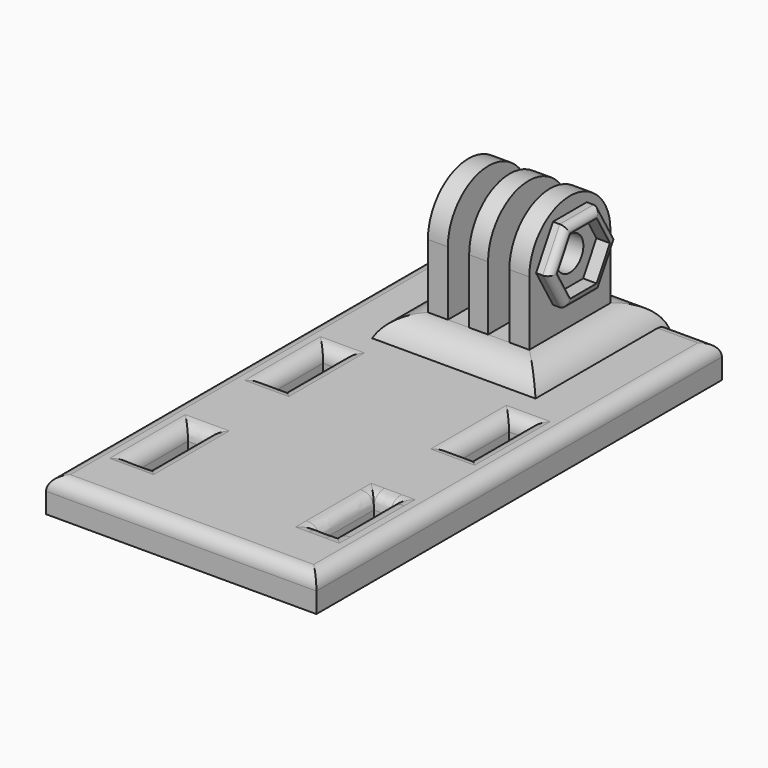
from build123d import *

# Parameters (mm, degrees)
F0_W           = 15
F0_H           = 3
F1_DEPTH       = 15
F2_DEPTH       = 3
F3_DEPTH       = 3
F4_DEPTH       = 2
F5_DEPTH       = 3
F6_DEPTH       = 12
F7_D           = 5
F7_DEPTH       = 15
F7_TIP         = 1.5021515476
F9_W           = 3.15
F9_H           = 15
F10_DEPTH      = 17
F11_R          = 1
F12_W          = 12.5
F12_H          = 12.5
F13_DEPTH      = 5
F14_T1_DEPTH   = 2.5
F14_T3_DEPTH   = 10
F14_T9_DEPTH   = 15
F14_T13_DEPTH  = 7.5
F14_T20_DEPTH  = 7.5
F14_T24_DEPTH  = 15
F14_T31_DEPTH  = 15
F14_T35_DEPTH  = 7.5
F14_T42_DEPTH  = 15
F14_T46_DEPTH  = 7.5
F15_R          = 2
F17_W          = 20
F17_H          = 12.5
F17_W_2        = 5
F18_DEPTH      = 3
F18_DEPTH_BACK = 2
F19_R          = 4.99999


# Not quite as in the source:
# - a fillet or chamfer that OpenCascade refuses, or shapes differently, is made with other operations: its cross-section is extruded or revolved along the edge and cut away or added
# - a fillet or chamfer is up to 0.001 mm smaller than in the source, because OpenCascade refuses the exact size


with BuildPart() as f1:
    # F0 (on Right) → F1 (new body)
    with BuildSketch(Plane.YZ):
        with Locations((0, 1.5)):
            Rectangle(F0_W, F0_H)
    extrude(amount=-F1_DEPTH)

    # F0 (on Right) → F2 (join)
    with BuildSketch(Plane.YZ):
        with BuildLine():
            Line((-7.5, 12.5), (-7.5, 3))
            Line((-7.5, 3), (7.5, 3))
            Line((7.5, 3), (7.5, 12.5))
            ThreePointArc((7.5, 12.5), (0, 20), (-7.5, 12.5))
        make_face()
        Polygon((-6.25, 12.5), (-3.125, 17.9126587737), (3.125, 17.9126587737), (6.25, 12.5), (3.125, 7.0873412263), (-3.125, 7.0873412263), align=None, mode=Mode.SUBTRACT)
    extrude(amount=-F2_DEPTH)

    # F0 (on Right) → F3 (join)
    with BuildSketch(Plane.YZ):
        Polygon((3.125, 17.9126587737), (-3.125, 17.9126587737), (-6.25, 12.5), (-3.125, 7.0873412263), (3.125, 7.0873412263), (6.25, 12.5), align=None)
        Polygon((-4.9074772881, 12.5), (-2.4537386441, 16.75), (2.4537386441, 16.75), (4.9074772881, 12.5), (2.4537386441, 8.25), (-2.4537386441, 8.25), align=None, mode=Mode.SUBTRACT)
    extrude(amount=-F3_DEPTH)

    # F0 (on Right) → F4 (join)
    with BuildSketch(Plane.YZ):
        Polygon((3.125, 17.9126587737), (-3.125, 17.9126587737), (-6.25, 12.5), (-3.125, 7.0873412263), (3.125, 7.0873412263), (6.25, 12.5), align=None)
        Polygon((-4.9074772881, 12.5), (-2.4537386441, 16.75), (2.4537386441, 16.75), (4.9074772881, 12.5), (2.4537386441, 8.25), (-2.4537386441, 8.25), align=None, mode=Mode.SUBTRACT)
    extrude(amount=F4_DEPTH)

    # F0 (on Right) → F5 (join)
    with BuildSketch(Plane.YZ):
        Polygon((2.4537386441, 16.75), (-2.4537386441, 16.75), (-4.9074772881, 12.5), (-2.4537386441, 8.25), (2.4537386441, 8.25), (4.9074772881, 12.5), align=None)
    extrude(amount=-F5_DEPTH)

    # F6 (add): a face of the model
    f6_faces = [f1.faces().sort_by_distance(p)[0] for p in [
        (-3, 0, 10.7862789639),
    ]]
    extrude(f6_faces, amount=F6_DEPTH)

    # F7
    with Locations(Plane.YZ):
        with Locations((0, 12.5)):
            Hole(F7_D / 2, depth=F7_DEPTH)
            with Locations((0, 0, -(F7_DEPTH + F7_TIP / 2))):  # 118° drill point
                Cone(0, F7_D / 2, F7_TIP, mode=Mode.SUBTRACT)

    # F9 (on offset) → F10 (cut)
    with BuildSketch(Plane.XY.offset(20)):
        with Locations((-10.475, 0)):
            Rectangle(F9_W, F9_H)
        with Locations((-4.525, 0)):
            Rectangle(F9_W, F9_H)
    extrude(amount=-F10_DEPTH, mode=Mode.SUBTRACT)

    # F11
    f11_edges = [f1.edges().sort_by_distance(p)[0] for p in [
        (2, -4.6875, 9.793671),
        (2, 0, 7.087341),
        (2, -4.6875, 15.206329),
        (2, 0, 17.912659),
        (2, 4.6875, 15.206329),
        (2, 4.6875, 9.793671),
    ]]
    fillet(f11_edges, radius=F11_R)


with BuildPart() as f13:
    # F12 (on face) → F13 (new body)
    with BuildSketch(Plane(origin=(0, 0, 0), x_dir=(1, 0, 0), z_dir=(0, 0, -1))):
        Polygon((-27.5, -12.5), (0, -12.5), (0, 0), (0, 62.5), (-20, 62.5), (-20, 52.5), (-20, 42.5), (-20, 27.5), (-20, 17.5), (-22.5, 17.5), (-27.5, 17.5), (-27.5, 0), align=None)
        with Locations((6.25, -6.25)):
            Rectangle(F12_W, F12_H)
        Polygon((0, 62.5), (0, 0), (12.5, 0), (12.5, 17.5), (7.5, 17.5), (5, 17.5), (5, 27.5), (5, 42.5), (5, 52.5), (5, 62.5), align=None)
        Polygon((-27.5, 42.5), (-27.5, 17.5), (-22.5, 17.5), (-22.5, 27.5), (-20, 27.5), (-20, 42.5), (-22.5, 42.5), align=None)
        Polygon((-20, 52.5), (-20, 62.5), (-27.5, 62.5), (-27.5, 42.5), (-22.5, 42.5), (-22.5, 52.5), align=None)
        Polygon((12.5, 62.5), (5, 62.5), (5, 52.5), (7.5, 52.5), (12.5, 52.5), align=None)
        Polygon((7.5, 17.5), (12.5, 17.5), (12.5, 52.5), (7.5, 52.5), (7.5, 42.5), (5, 42.5), (5, 27.5), (7.5, 27.5), align=None)
    extrude(amount=F13_DEPTH)

    # F14: fillet of radius 2 on 4 edges, made by hand

    # F14_s2 → F14_t1 (cut)
    with BuildSketch(Plane.YZ.offset(5)):
        with BuildLine():
            add(Edge.make_bspline(
                [(-52.5, -2), (-52.5, 0), (-54.5, 0)],
                knots=[0, 0, 0, 1, 1, 1], degree=2, weights=[1, 1, 1]))
            Line((-54.5, 0), (-52.5, 0))
            Line((-52.5, 0), (-52.5, -2))
        make_face()
        with BuildLine():
            add(Edge.make_bspline(
                [(-42.5, -2), (-42.5, 0), (-40.5, 0)],
                knots=[0, 0, 0, 1, 1, 1], degree=2, weights=[1, 1, 1]))
            Line((-40.5, 0), (-42.5, 0))
            Line((-42.5, 0), (-42.5, -2))
        make_face()
    extrude(amount=F14_T1_DEPTH, mode=Mode.SUBTRACT)

    # F14_s4 → F14_t3 (cut)
    with BuildSketch(Plane.XZ.offset(42.5)):
        with BuildLine():
            add(Edge.make_bspline(
                [(7.5, -2), (7.5, 0), (9.5, 0)],
                knots=[0, 0, 0, 1, 1, 1], degree=2, weights=[1, 1, 1]))
            Line((9.5, 0), (7.5, 0))
            Line((7.5, 0), (7.5, -2))
        make_face()
        with BuildLine():
            add(Edge.make_bspline(
                [(5, -2), (5, 0), (3, 0)],
                knots=[0, 0, 0, 1, 1, 1], degree=2, weights=[1, 1, 1]))
            Line((3, 0), (5, 0))
            Line((5, 0), (5, -2))
        make_face()
    extrude(amount=F14_T3_DEPTH, mode=Mode.SUBTRACT)


with BuildPart() as f14_tool7:
    # F14_s8 → F14_t9 (new body)
    with BuildSketch(Plane.XZ.offset(42.5)):
        with BuildLine():
            add(Edge.make_bspline(
                [(5, -2), (5, 0), (3, 0)],
                knots=[0, 0, 0, 1, 1, 1], degree=2, weights=[1, 1, 1]))
            Line((3, 0), (5, 0))
            Line((5, 0), (5, -2))
        make_face()
    extrude(amount=F14_T9_DEPTH)

    split(bisect_by=Plane.XZ.offset(52.5), keep=Keep.TOP)


with BuildPart() as f14_tool11:
    # F14_s12 → F14_t13 (new body)
    with BuildSketch(Plane.YZ):
        with BuildLine():
            add(Edge.make_bspline(
                [(-52.5, -2), (-52.5, 0), (-54.5, 0)],
                knots=[0, 0, 0, 1, 1, 1], degree=2, weights=[1, 1, 1]))
            Line((-54.5, 0), (-52.5, 0))
            Line((-52.5, 0), (-52.5, -2))
        make_face()
    extrude(amount=F14_T13_DEPTH)

    split(bisect_by=Plane.YZ.offset(5), keep=Keep.BOTTOM)


with BuildPart() as f14_tool7_1:
    add(f14_tool7.part)

    # F14_t15: intersect F14_tool11
    add(f14_tool11.part, mode=Mode.INTERSECT)


with BuildPart() as f13_1:
    add(f13.part)

    # F14_t5: cut F14_tool7
    add(f14_tool7_1.part, mode=Mode.SUBTRACT)


with BuildPart() as f14_tool18:
    # F14_s19 → F14_t20 (new body)
    with BuildSketch(Plane.YZ.offset(5)):
        with BuildLine():
            add(Edge.make_bspline(
                [(-52.5, -2), (-52.5, 0), (-54.5, 0)],
                knots=[0, 0, 0, 1, 1, 1], degree=2, weights=[1, 1, 1]))
            Line((-54.5, 0), (-52.5, 0))
            Line((-52.5, 0), (-52.5, -2))
        make_face()
    extrude(amount=F14_T20_DEPTH)

    split(bisect_by=Plane.YZ.offset(7.5), keep=Keep.TOP)


with BuildPart() as f14_tool22:
    # F14_s23 → F14_t24 (new body)
    with BuildSketch(Plane.XZ.offset(57.5)):
        with BuildLine():
            add(Edge.make_bspline(
                [(7.5, -2), (7.5, 0), (9.5, 0)],
                knots=[0, 0, 0, 1, 1, 1], degree=2, weights=[1, 1, 1]))
            Line((9.5, 0), (7.5, 0))
            Line((7.5, 0), (7.5, -2))
        make_face()
    extrude(amount=-F14_T24_DEPTH)

    split(bisect_by=Plane.XZ.offset(52.5), keep=Keep.TOP)


with BuildPart() as f14_tool18_1:
    add(f14_tool18.part)

    # F14_t26: intersect F14_tool22
    add(f14_tool22.part, mode=Mode.INTERSECT)


with BuildPart() as f13_2:
    add(f13_1.part)

    # F14_t16: cut F14_tool18
    add(f14_tool18_1.part, mode=Mode.SUBTRACT)


with BuildPart() as f14_tool29:
    # F14_s30 → F14_t31 (new body)
    with BuildSketch(Plane.XZ.offset(52.5)):
        with BuildLine():
            add(Edge.make_bspline(
                [(7.5, -2), (7.5, 0), (9.5, 0)],
                knots=[0, 0, 0, 1, 1, 1], degree=2, weights=[1, 1, 1]))
            Line((9.5, 0), (7.5, 0))
            Line((7.5, 0), (7.5, -2))
        make_face()
    extrude(amount=-F14_T31_DEPTH)

    split(bisect_by=Plane.XZ.offset(42.5), keep=Keep.BOTTOM)


with BuildPart() as f14_tool33:
    # F14_s34 → F14_t35 (new body)
    with BuildSketch(Plane.YZ.offset(12.5)):
        with BuildLine():
            add(Edge.make_bspline(
                [(-42.5, -2), (-42.5, 0), (-40.5, 0)],
                knots=[0, 0, 0, 1, 1, 1], degree=2, weights=[1, 1, 1]))
            Line((-40.5, 0), (-42.5, 0))
            Line((-42.5, 0), (-42.5, -2))
        make_face()
    extrude(amount=-F14_T35_DEPTH)

    split(bisect_by=Plane.YZ.offset(7.5), keep=Keep.TOP)


with BuildPart() as f14_tool29_1:
    add(f14_tool29.part)

    # F14_t37: intersect F14_tool33
    add(f14_tool33.part, mode=Mode.INTERSECT)


with BuildPart() as f13_3:
    add(f13_2.part)

    # F14_t27: cut F14_tool29
    add(f14_tool29_1.part, mode=Mode.SUBTRACT)


with BuildPart() as f14_tool40:
    # F14_s41 → F14_t42 (new body)
    with BuildSketch(Plane.XZ.offset(37.5)):
        with BuildLine():
            add(Edge.make_bspline(
                [(5, -2), (5, 0), (3, 0)],
                knots=[0, 0, 0, 1, 1, 1], degree=2, weights=[1, 1, 1]))
            Line((3, 0), (5, 0))
            Line((5, 0), (5, -2))
        make_face()
    extrude(amount=F14_T42_DEPTH)

    split(bisect_by=Plane.XZ.offset(42.5), keep=Keep.BOTTOM)


with BuildPart() as f14_tool44:
    # F14_s45 → F14_t46 (new body)
    with BuildSketch(Plane.YZ.offset(7.5)):
        with BuildLine():
            add(Edge.make_bspline(
                [(-42.5, -2), (-42.5, 0), (-40.5, 0)],
                knots=[0, 0, 0, 1, 1, 1], degree=2, weights=[1, 1, 1]))
            Line((-40.5, 0), (-42.5, 0))
            Line((-42.5, 0), (-42.5, -2))
        make_face()
    extrude(amount=-F14_T46_DEPTH)

    split(bisect_by=Plane.YZ.offset(5), keep=Keep.BOTTOM)


with BuildPart() as f14_tool40_1:
    add(f14_tool40.part)

    # F14_t48: intersect F14_tool44
    add(f14_tool44.part, mode=Mode.INTERSECT)


with BuildPart() as f13_4:
    add(f13_3.part)

    # F14_t38: cut F14_tool40
    add(f14_tool40_1.part, mode=Mode.SUBTRACT)

    # F15
    f15_edges = [f13_4.edges().sort_by_distance(p)[0] for p in [
        (-22.5, -47.5, 0),
        (-21.25, -52.5, 0),
        (-20, -47.5, 0),
        (-21.25, -42.5, 0),
        (5, -22.5, 0),
        (6.25, -27.5, 0),
        (7.5, -22.5, 0),
        (6.25, -17.5, 0),
        (-20, -22.5, 0),
        (-21.25, -27.5, 0),
        (-22.5, -22.5, 0),
        (-21.25, -17.5, 0),
        (12.5, -25, 0),
        (-27.5, -25, 0),
        (-7.5, 12.5, 0),
        (-7.5, -62.5, 0),
    ]]
    fillet(f15_edges, radius=F15_R)


with BuildPart() as f18:
    # F17 (on face) → F18 (new body, two sides)
    with BuildSketch(Plane.XY) as f18_sk:
        with Locations((-10, -6.25)):
            Rectangle(F17_W, F17_H)
        with Locations((2.5, -6.25)):
            Rectangle(F17_W_2, F17_H)
        with Locations((-10, 6.25)):
            Rectangle(F17_W, F17_H)
        with Locations((2.5, 6.25)):
            Rectangle(F17_W_2, F17_H)
    extrude(amount=F18_DEPTH)
    extrude(f18_sk.sketch, amount=-F18_DEPTH_BACK)

    # F19 (radius 5 in the source; OpenCascade refuses exactly that, so slightly less here)
    f19_edges = [f18.edges().sort_by_distance(p)[0] for p in [
        (5, 0, 3),
        (-7.5, -12.5, 3),
        (-20, 0, 3),
        (-7.5, 12.5, 3),
    ]]
    fillet(f19_edges, radius=F19_R)


solid = Compound([f1.part, f13_4.part, f18.part])
